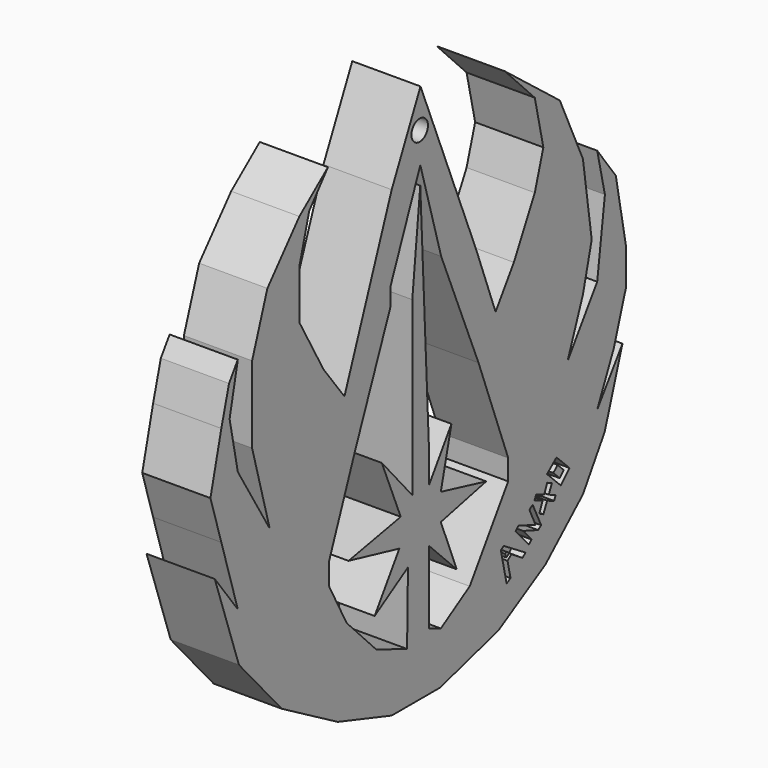
from build123d import *

# Parameters (mm, degrees)
F1_DEPTH = 5
F2_R     = 0.7543712854
F3_DEPTH = 5
F5_DEPTH = 1


# Not quite as in the source:
# - a feature names something its author has since deleted; it is built from what else it names


with BuildPart() as f1:
    # F0 (on Right) → F1 (new body)
    with BuildSketch(Plane.YZ):
        Polygon((-18.8395921141, 32.0152118802), (-23.9240508527, 44.5727854967), (-23.9400436678, 39.4980984787), (-22.0310017467, 32.8367650509), (-18.6073519289, 24.5797261596), (-15.8885698766, 17.3296425492), (-15.8885698766, 15.8192086965), (-19.4129161537, 10.4823429137), (-22.0608360687, 8.8354363138), (-22.1316963434, 5.0447816029), (-16.7948305607, 6.5552145243), (-12.4649200588, 9.0726036578), (-9.0412702411, 12.1941678226), (-7.0434443557, 15.421631052), (-5.4162289016, 20.4512067139), (-7.732226979, 17.128251493), (-6.221793592, 20.4512067139), (-5.1141423173, 23.8748565316), (-5.1141423173, 26.6943331808), (-6.0204025358, 31.5277203918), (-7.732226979, 33.8437184691), (-7.0273578167, 30.722156167), (-7.732226979, 25.3852903843), (-10.4510085657, 21.3574655354), (-9.0412702411, 25.0832028687), (-8.2357050851, 28.3054616302), (-9.0412702411, 33.8437184691), (-11.1558772624, 38.4757146239), (-16.1906573921, 42.4028448761), (-13.4509364143, 39.5833663642), (-12.666311115, 36.0590219498), (-13.4509364143, 33.4521867335), (-15.3669025749, 29.7400020063), (-17.0433744788, 27.2252950817), align=None)
        Polygon((-23.9400436678, 39.4980984787), (-23.9240508527, 44.5727854967), (-26.5623033047, 38.9791950583), (-30.8922119439, 27.3992009461), (-32.8054279089, 29.9165919423), (-35.0207313895, 33.8437184691), (-35.0207313895, 37.4687612057), (-34.114472568, 40.6910181046), (-32.4026457965, 42.8056269884), (-35.0207313895, 40.6910181046), (-37.9520406538, 37.2414154054), (-39.350643754, 33.1388488412), (-39.350643754, 27.4998974055), (-37.7395115793, 21.659553051), (-40.6596846879, 26.492940262), (-41.4149016142, 30.2186775953), (-40.6596846879, 33.7430238724), (-41.4652489126, 32.5346775353), (-42.1701185405, 29.9165919423), (-43.169213802, 25.8295247582), (-42.1701185405, 22.5658137351), (-40.6596846879, 17.6317300647), (-42.7742935717, 20.4512067139), (-40.5589900911, 14.0066882595), (-36.631859839, 9.5760822296), (-31.5034037335, 6.6433727204), (-26.5623033047, 5.0447816029), (-25.1525640488, 8.7705180049), (-27.9720406979, 9.8781688139), (-30.6908208877, 12.697645463), (-32.3019511998, 15.7185140997), (-32.3019511998, 17.3296425492), (-29.885256663, 23.572769016), (-26.6505166424, 31.5225556516), (-26.6505166424, 32.8367650509), align=None)
        Polygon((-22.1316963434, 5.0447816029), (-22.0608360687, 8.8354363138), (-23.1386516243, 9.2739956453), (-23.1386516243, 14.6031556651), (-25.0721577589, 14.0031509837), (-25.1525640488, 8.7705180049), (-26.5623033047, 5.0447816029), align=None)
        Polygon((-23.1386516243, 20.699724555), (-23.9442177117, 38.1736308336), (-24.6739685535, 31.1146955937), (-24.6739685535, 24.4254041463), (-24.6739685535, 18.4981841594), (-27.4682287127, 21.715817973), (-25.7342918677, 17.5339697332), (-30.516512692, 16.6353452951), (-25.8594118059, 15.5345760286), (-28.1243625509, 12.1047943952), (-25.0721577589, 14.0031509837), (-23.1386516243, 14.6031556651), (-20.6095892936, 12.0629183948), (-22.0608360687, 15.7039240003), (-17.9000031203, 16.6353452951), (-22.0608360687, 17.6514387131), (-21.0862746716, 21.6422008803), (-23.1386516243, 18.5343166173), align=None)
    extrude(amount=F1_DEPTH)

    # F2 (on face) → F3 (cut)
    with BuildSketch(Plane.YZ.offset(5)):
        with Locations((-23.9965710789, 41.7759902775)):
            Circle(F2_R)
    extrude(amount=-F3_DEPTH, mode=Mode.SUBTRACT)

    # F4 (on face) → F5 (cut)
    with BuildSketch(Plane.YZ.offset(5)):
        Polygon((-16.5610130304, 11.6452822793), (-16.0314254463, 9.2795155942), (-15.6742927399, 9.4880603932), (-15.9501638263, 10.7204280794), (-15.5902979895, 10.9956199303), (-14.5742027089, 10.3393923491), (-14.309595339, 10.5828316882), (-16.2962192383, 11.8211973459), align=None)
        Polygon((-15.7808158547, 11.1649697646), (-16.056008637, 10.9638674185), (-16.1724351346, 11.2602282315), (-16.0208165755, 11.319792172), align=None, mode=Mode.SUBTRACT)
        Polygon((-15.2138965204, 12.3287355527), (-14.0034528449, 10.9638674185), (-13.7453717467, 11.1927486014), (-14.5170884397, 12.0629183948), (-13.149023056, 11.563308537), (-12.8642125055, 11.759115383), (-13.6474408209, 13.3967734873), (-13.9450938452, 13.192137459), (-13.3804315701, 11.9905229658), (-14.9350901603, 12.5759970916), align=None)
        Polygon((-13.31801555, 13.93365104), (-13.4715074673, 13.610381633), (-12.7293292628, 13.2944049069), (-12.5892657792, 13.6233913674), align=None)
        Polygon((-12.5892657792, 13.6233913674), (-12.7293292628, 13.2944049069), (-12.3227360628, 13.1213009442), (-12.1738159695, 13.4465167705), align=None)
        Polygon((-12.3227360628, 13.1213009442), (-12.7293292628, 13.2944049069), (-13.0343568597, 12.5779444352), (-12.6627200979, 12.3788343877), align=None)
        Polygon((-12.1738159695, 13.4465167705), (-12.3227360628, 13.1213009442), (-11.6736432537, 12.8449546173), (-11.5335797702, 13.1739410778), align=None)
        Polygon((-12.3115735045, 14.2756455901), (-12.5892657792, 13.6233913674), (-12.1738159695, 13.4465167705), (-11.8785644276, 14.0912952688), align=None)
        Polygon((-11.4597871365, 15.568957784), (-12.3322671279, 14.8386247456), (-11.0684223473, 13.5925812647), (-10.2732402928, 14.3991234958), align=None)
        Polygon((-11.7448461242, 14.678419102), (-11.3710323349, 15.0522328913), (-10.8014121652, 14.4826127216), (-11.1752259545, 14.1087989323), align=None, mode=Mode.SUBTRACT)
    extrude(amount=-F5_DEPTH, mode=Mode.SUBTRACT)


solid = f1.part
